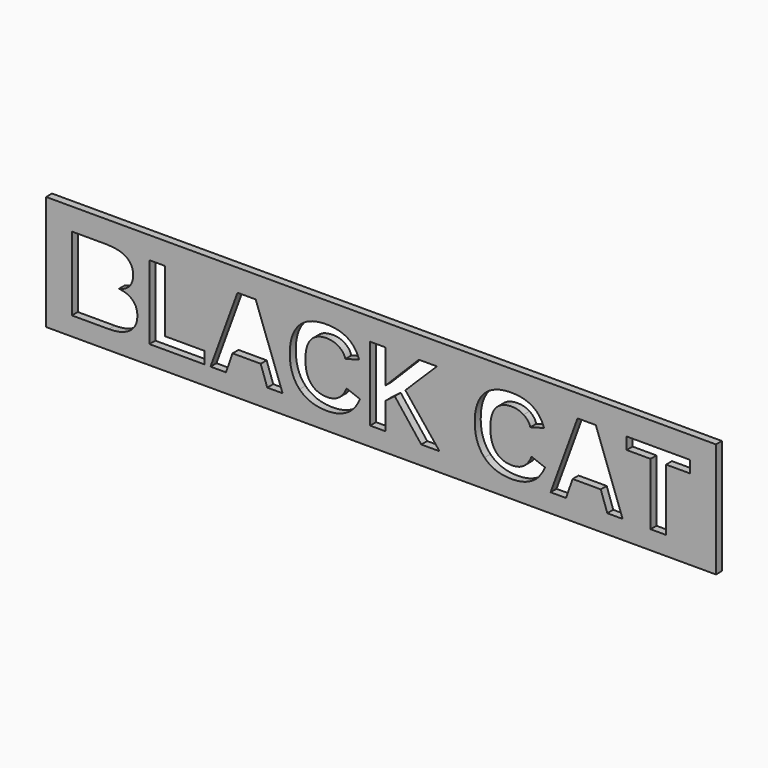
from build123d import *

# Parameters (mm, degrees)
F0_W     = 180
F0_H     = 30.7765754297
F1_DEPTH = 2


with BuildPart() as f1:
    # F0 (on Front) → F1 (new body)
    with BuildSketch(Plane.XZ):
        with Locations((37.3380143768, 10.3882877148)):
            Rectangle(F0_W, F0_H)
        with BuildLine():
            add(Edge.make_bspline(
                [(-29.3945604163, 8.9251803522), (-28.1343492982, 7.6920220666), (-28.1343492982, 5.6630596223)],
                knots=[0, 0, 0, 1, 1, 1], degree=2))
            add(Edge.make_bspline(
                [(-28.1343492982, 5.6630596223), (-28.1343492982, 2.9577763633), (-30.1633117425, 1.4788881816)],
                knots=[0, 0, 0, 1, 1, 1], degree=2))
            add(Edge.make_bspline(
                [(-30.1633117425, 1.4788881816), (-32.1922741868, 0), (-35.7993185322, 0)],
                knots=[0, 0, 0, 1, 1, 1], degree=2))
            Line((-35.7993185322, 0), (-45.7322168984, 0))
            Line((-45.7322168984, 0), (-45.7322168984, 19.8522703161))
            Line((-45.7322168984, 19.8522703161), (-36.6424651479, 19.8522703161))
            add(Edge.make_bspline(
                [(-36.6424651479, 19.8522703161), (-33.0083679699, 19.8522703161), (-31.1417225212, 18.592059198)],
                knots=[0, 0, 0, 1, 1, 1], degree=2))
            add(Edge.make_bspline(
                [(-31.1417225212, 18.592059198), (-29.2750770724, 17.3318480798), (-29.2750770724, 14.8655315086)],
                knots=[0, 0, 0, 1, 1, 1], degree=2))
            add(Edge.make_bspline(
                [(-29.2750770724, 14.8655315086), (-29.2750770724, 13.1747294717), (-30.2106541995, 12.0114576703)],
                knots=[0, 0, 0, 1, 1, 1], degree=2))
            add(Edge.make_bspline(
                [(-30.2106541995, 12.0114576703), (-31.1462313266, 10.8481858689), (-33.0624736351, 10.44239338)],
                knots=[0, 0, 0, 1, 1, 1], degree=2))
            add(Edge.make_bspline(
                [(-33.0624736351, 10.44239338), (-30.6547715345, 10.1583386378), (-29.3945604163, 8.9251803522)],
                knots=[0, 0, 0, 1, 1, 1], degree=2))
        make_face(mode=Mode.SUBTRACT)
        Polygon((-10.0810923493, 0), (-24.8925181927, 0), (-24.8925181927, 19.8522703161), (-20.7353995846, 19.8522703161), (-20.7353995846, 3.2147782729), (-10.0810923493, 3.2147782729), align=None, mode=Mode.SUBTRACT)
        Polygon((10.8803441031, 0), (6.7683135493, 0), (5.0053706255, 5.0724061108), (-2.5604048891, 5.0724061108), (-4.3233478129, 0), (-8.480466421, 0), (-1.2348160921, 19.8522703161), (3.6662554122, 19.8522703161), align=None, mode=Mode.SUBTRACT)
        with BuildLine():
            add(Edge.make_bspline(
                [(18.5114972964, 4.792860174), (20.0106751024, 2.9893380013), (22.8422049136, 2.9893380013)],
                knots=[0, 0, 0, 1, 1, 1], degree=2))
            add(Edge.make_bspline(
                [(22.8422049136, 2.9893380013), (26.6070574491, 2.9893380013), (28.0724192145, 6.7632081477)],
                knots=[0, 0, 0, 1, 1, 1], degree=2))
            Line((28.0724192145, 6.7632081477), (31.6929899762, 5.3970401018))
            add(Edge.make_bspline(
                [(31.6929899762, 5.3970401018), (30.5252093694, 2.5204222364), (28.2617890426, 1.1181837471)],
                knots=[0, 0, 0, 1, 1, 1], degree=2))
            add(Edge.make_bspline(
                [(28.2617890426, 1.1181837471), (25.9983687158, -0.2840547422), (22.8422049136, -0.2840547422)],
                knots=[0, 0, 0, 1, 1, 1], degree=2))
            add(Edge.make_bspline(
                [(22.8422049136, -0.2840547422), (18.053853545, -0.2840547422), (15.4410007973, 2.4302461277)],
                knots=[0, 0, 0, 1, 1, 1], degree=2))
            add(Edge.make_bspline(
                [(15.4410007973, 2.4302461277), (12.8281480496, 5.1445469977), (12.8281480496, 10.0185656694)],
                knots=[0, 0, 0, 1, 1, 1], degree=2))
            add(Edge.make_bspline(
                [(12.8281480496, 10.0185656694), (12.8281480496, 14.9061107575), (15.348570286, 17.5279811161)],
                knots=[0, 0, 0, 1, 1, 1], degree=2))
            add(Edge.make_bspline(
                [(15.348570286, 17.5279811161), (17.8689925223, 20.1498514746), (22.6618526963, 20.1498514746)],
                knots=[0, 0, 0, 1, 1, 1], degree=2))
            add(Edge.make_bspline(
                [(22.6618526963, 20.1498514746), (26.156176906, 20.1498514746), (28.3542195539, 18.7476129854)],
                knots=[0, 0, 0, 1, 1, 1], degree=2))
            add(Edge.make_bspline(
                [(28.3542195539, 18.7476129854), (30.5522622019, 17.3453744961), (31.440496872, 14.6265648207)],
                knots=[0, 0, 0, 1, 1, 1], degree=2))
            Line((31.440496872, 14.6265648207), (27.774838056, 13.6256100149))
            add(Edge.make_bspline(
                [(27.774838056, 13.6256100149), (27.3104310965, 15.1180246128), (25.9510262588, 15.9994960747)],
                knots=[0, 0, 0, 1, 1, 1], degree=2))
            add(Edge.make_bspline(
                [(25.9510262588, 15.9994960747), (24.5916214211, 16.8809675366), (22.7475199995, 16.8809675366)],
                knots=[0, 0, 0, 1, 1, 1], degree=2))
            add(Edge.make_bspline(
                [(22.7475199995, 16.8809675366), (19.9295166047, 16.8809675366), (18.4709180475, 15.1338054318)],
                knots=[0, 0, 0, 1, 1, 1], degree=2))
            add(Edge.make_bspline(
                [(18.4709180475, 15.1338054318), (17.0123194903, 13.386643327), (17.0123194903, 10.0185656694)],
                knots=[0, 0, 0, 1, 1, 1], degree=2))
            add(Edge.make_bspline(
                [(17.0123194903, 10.0185656694), (17.0123194903, 6.5963823467), (18.5114972964, 4.792860174)],
                knots=[0, 0, 0, 1, 1, 1], degree=2))
        make_face(mode=Mode.SUBTRACT)
        Polygon((53.055710112, 0), (48.1501298022, 0), (41.0217084145, 9.1168045831), (38.5689182597, 7.2411415234), (38.5689182597, 0), (34.4117996515, 0), (34.4117996515, 19.8522703161), (38.5689182597, 19.8522703161), (38.5689182597, 10.8481858689), (47.5143882363, 19.8522703161), (52.3613540755, 19.8522703161), (43.8802910583, 11.4568746022), align=None, mode=Mode.SUBTRACT)
        with BuildLine():
            add(Edge.make_bspline(
                [(68.2075507655, 4.792860174), (69.7067285716, 2.9893380013), (72.5382583827, 2.9893380013)],
                knots=[0, 0, 0, 1, 1, 1], degree=2))
            add(Edge.make_bspline(
                [(72.5382583827, 2.9893380013), (76.3031109183, 2.9893380013), (77.7684726836, 6.7632081477)],
                knots=[0, 0, 0, 1, 1, 1], degree=2))
            Line((77.7684726836, 6.7632081477), (81.3890434453, 5.3970401018))
            add(Edge.make_bspline(
                [(81.3890434453, 5.3970401018), (80.2212628385, 2.5204222364), (77.9578425117, 1.1181837471)],
                knots=[0, 0, 0, 1, 1, 1], degree=2))
            add(Edge.make_bspline(
                [(77.9578425117, 1.1181837471), (75.694422185, -0.2840547422), (72.5382583827, -0.2840547422)],
                knots=[0, 0, 0, 1, 1, 1], degree=2))
            add(Edge.make_bspline(
                [(72.5382583827, -0.2840547422), (67.7499070142, -0.2840547422), (65.1370542664, 2.4302461277)],
                knots=[0, 0, 0, 1, 1, 1], degree=2))
            add(Edge.make_bspline(
                [(65.1370542664, 2.4302461277), (62.5242015187, 5.1445469977), (62.5242015187, 10.0185656694)],
                knots=[0, 0, 0, 1, 1, 1], degree=2))
            add(Edge.make_bspline(
                [(62.5242015187, 10.0185656694), (62.5242015187, 14.9061107575), (65.0446237551, 17.5279811161)],
                knots=[0, 0, 0, 1, 1, 1], degree=2))
            add(Edge.make_bspline(
                [(65.0446237551, 17.5279811161), (67.5650459915, 20.1498514746), (72.3579061654, 20.1498514746)],
                knots=[0, 0, 0, 1, 1, 1], degree=2))
            add(Edge.make_bspline(
                [(72.3579061654, 20.1498514746), (75.8522303751, 20.1498514746), (78.0502730231, 18.7476129854)],
                knots=[0, 0, 0, 1, 1, 1], degree=2))
            add(Edge.make_bspline(
                [(78.0502730231, 18.7476129854), (80.2483156711, 17.3453744961), (81.1365503411, 14.6265648207)],
                knots=[0, 0, 0, 1, 1, 1], degree=2))
            Line((81.1365503411, 14.6265648207), (77.4708915251, 13.6256100149))
            add(Edge.make_bspline(
                [(77.4708915251, 13.6256100149), (77.0064845656, 15.1180246128), (75.6470797279, 15.9994960747)],
                knots=[0, 0, 0, 1, 1, 1], degree=2))
            add(Edge.make_bspline(
                [(75.6470797279, 15.9994960747), (74.2876748903, 16.8809675366), (72.4435734687, 16.8809675366)],
                knots=[0, 0, 0, 1, 1, 1], degree=2))
            add(Edge.make_bspline(
                [(72.4435734687, 16.8809675366), (69.6255700738, 16.8809675366), (68.1669715166, 15.1338054318)],
                knots=[0, 0, 0, 1, 1, 1], degree=2))
            add(Edge.make_bspline(
                [(68.1669715166, 15.1338054318), (66.7083729594, 13.386643327), (66.7083729594, 10.0185656694)],
                knots=[0, 0, 0, 1, 1, 1], degree=2))
            add(Edge.make_bspline(
                [(66.7083729594, 10.0185656694), (66.7083729594, 6.5963823467), (68.2075507655, 4.792860174)],
                knots=[0, 0, 0, 1, 1, 1], degree=2))
        make_face(mode=Mode.SUBTRACT)
        Polygon((102.2557949836, 0), (98.1437644298, 0), (96.380821506, 5.0724061108), (88.8150459915, 5.0724061108), (87.0521030676, 0), (82.8949844595, 0), (90.1406347884, 19.8522703161), (95.0417062928, 19.8522703161), align=None, mode=Mode.SUBTRACT)
        Polygon((120.3361047651, 16.6420008487), (113.9110570248, 16.6420008487), (113.9110570248, 0), (109.7539384167, 0), (109.7539384167, 16.6420008487), (103.3424170927, 16.6420008487), (103.3424170927, 19.8522703161), (120.3361047651, 19.8522703161), align=None, mode=Mode.SUBTRACT)
    extrude(amount=F1_DEPTH)


solid = f1.part
